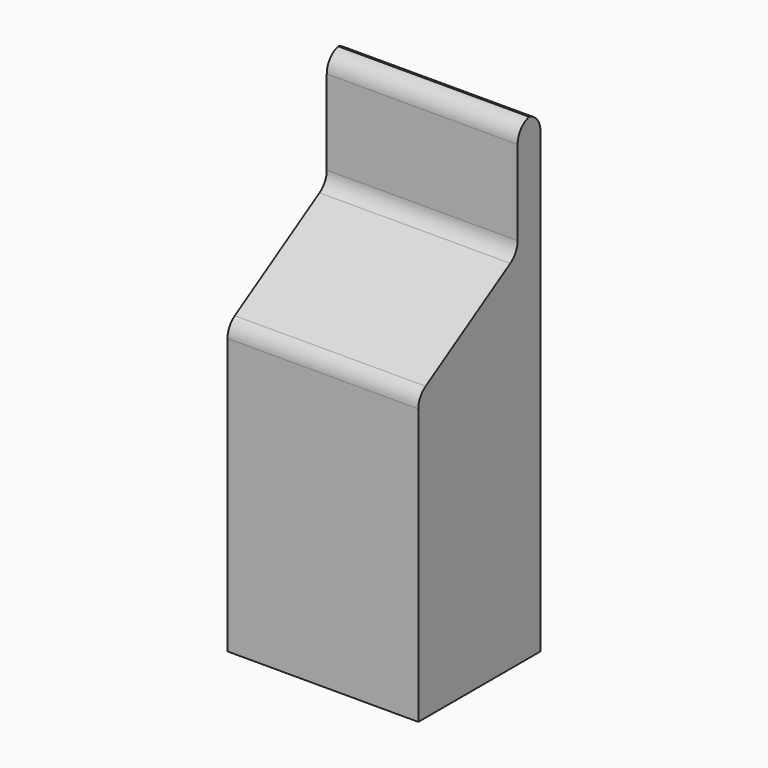
from build123d import *

# Parameters (mm, degrees)
F1_DEPTH    = 50
F2_T1_DEPTH = 50
F2_T3_DEPTH = 75
F2_T5_DEPTH = 63.9698798509


# Not quite as in the source:
# - a fillet or chamfer that OpenCascade refuses, or shapes differently, is made with other operations: its cross-section is extruded or revolved along the edge and cut away or added


with BuildPart() as f1:
    # F0 (on Right) → F1 (new body)
    with BuildSketch(Plane.YZ):
        Polygon((-32.5, 24.4166636232), (-32.5, -50.5833363768), (7.5, -50.5833363768), (7.5, 74.4166636232), (0, 74.4166636232), (0, 44.4166636232), align=None)
    extrude(amount=F1_DEPTH)

    # F2: fillet of radius 5 on 4 edges, made by hand

    # F2_s2 → F2_t1 (join)
    with BuildSketch(Plane.YZ):
        with BuildLine():
            ThreePointArc((-2.3795128717, 42.9523480098), (-0.6352299235, 44.7716270515), (0, 47.2106395933))
            Line((0, 47.2106395933), (0, 44.4166636232))
            Line((0, 44.4166636232), (-2.3795128717, 42.9523480098))
        make_face()
    extrude(amount=F2_T1_DEPTH)

    # F2_s4 → F2_t3 (cut)
    with BuildSketch(Plane.YZ.offset(-12.5)):
        with BuildLine():
            ThreePointArc((5, 74.4166636232), (1.4644660941, 72.9521975291), (0, 69.4166636232))
            Line((0, 69.4166636232), (0, 74.4166636232))
            Line((0, 74.4166636232), (5, 74.4166636232))
        make_face()
        with BuildLine():
            ThreePointArc((7.5, 69.4166636232), (6.0355339059, 72.9521975291), (2.5, 74.4166636232))
            Line((2.5, 74.4166636232), (7.5, 74.4166636232))
            Line((7.5, 74.4166636232), (7.5, 69.4166636232))
        make_face()
    extrude(amount=F2_T3_DEPTH, mode=Mode.SUBTRACT)

    # F2_s6 → F2_t5 (cut)
    with BuildSketch(Plane.YZ.offset(-6.9849399255)):
        with BuildLine():
            ThreePointArc((-30.1204871283, 25.8809792365), (-31.8647700765, 24.0617001948), (-32.5, 21.622687653))
            Line((-32.5, 21.622687653), (-32.5, 24.4166636232))
            Line((-32.5, 24.4166636232), (-30.1204871283, 25.8809792365))
        make_face()
    extrude(amount=F2_T5_DEPTH, mode=Mode.SUBTRACT)


solid = f1.part
